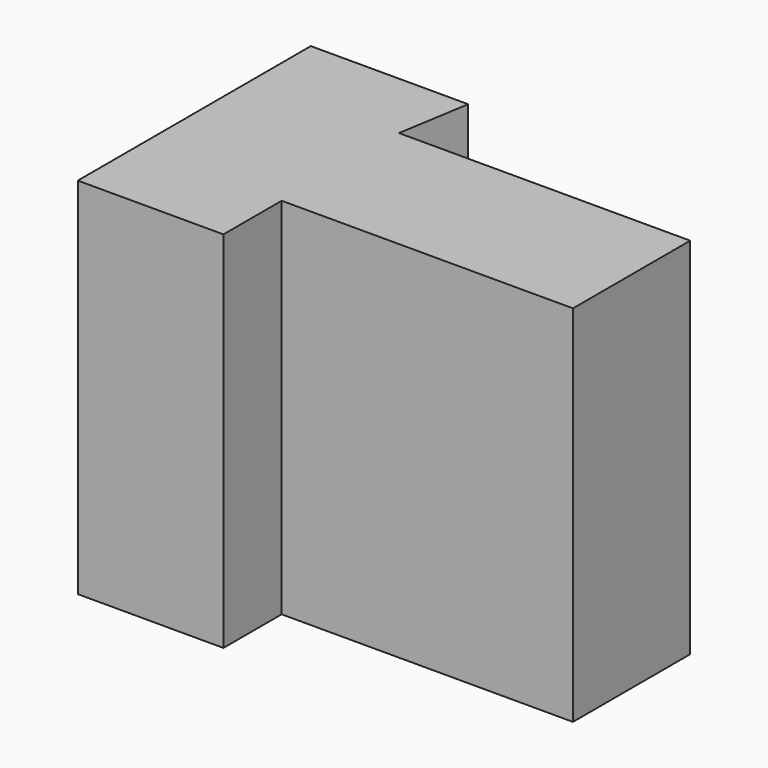
from build123d import *

# Parameters (mm, degrees)
F0_W     = 38.1
F0_H     = 31.75
F1_DEPTH = 25.4
F2_W     = 25.4
F2_H     = 6.35
F3_DEPTH = 25.4
F4_DEPTH = 6.35
F6_DEPTH = 31.75
F7_DEPTH = 57.15
F8_DEPTH = 25.4


with BuildPart() as f1:
    # F0 (on Front) → F1 (new body)
    with BuildSketch(Plane.XZ):
        with Locations((-40.7485894724, 15.875)):
            Rectangle(F0_W, F0_H)
    extrude(amount=F1_DEPTH)

    # F2 (on face) → F3 (cut)
    with BuildSketch(Plane.XY.offset(31.75)):
        with Locations((-34.3985894724, -22.225)):
            Rectangle(F2_W, F2_H)
    extrude(amount=-F3_DEPTH, mode=Mode.SUBTRACT)

    # F4 (cut): a face of the model
    f4_faces = [f1.faces().sort_by_distance(p)[0] for p in [
        (-34.3985894724, -22.225, 6.35),
    ]]
    extrude(f4_faces, amount=-F4_DEPTH, mode=Mode.SUBTRACT)

    # F5 (on face) → F6 (join)
    with BuildSketch(Plane.XY.offset(31.75)):
        Polygon((-47.0985894724, -6.2670672635), (-21.6985894724, -6.2670672635), (-21.6985894724, 0), (-46.0756682071, 0), align=None)
    extrude(amount=F6_DEPTH)

    # F7 (cut): a face of the model
    f7_faces = [f1.faces().sort_by_distance(p)[0] for p in [
        (-34.1446109127, -3.1549983853, 63.5),
    ]]
    extrude(f7_faces, amount=-F7_DEPTH, mode=Mode.SUBTRACT)

    # F8 (cut): a face of the model
    f8_faces = [f1.faces().sort_by_distance(p)[0] for p in [
        (-34.1446109127, -3.1549983853, 6.35),
    ]]
    extrude(f8_faces, amount=-F8_DEPTH, mode=Mode.SUBTRACT)


solid = f1.part
